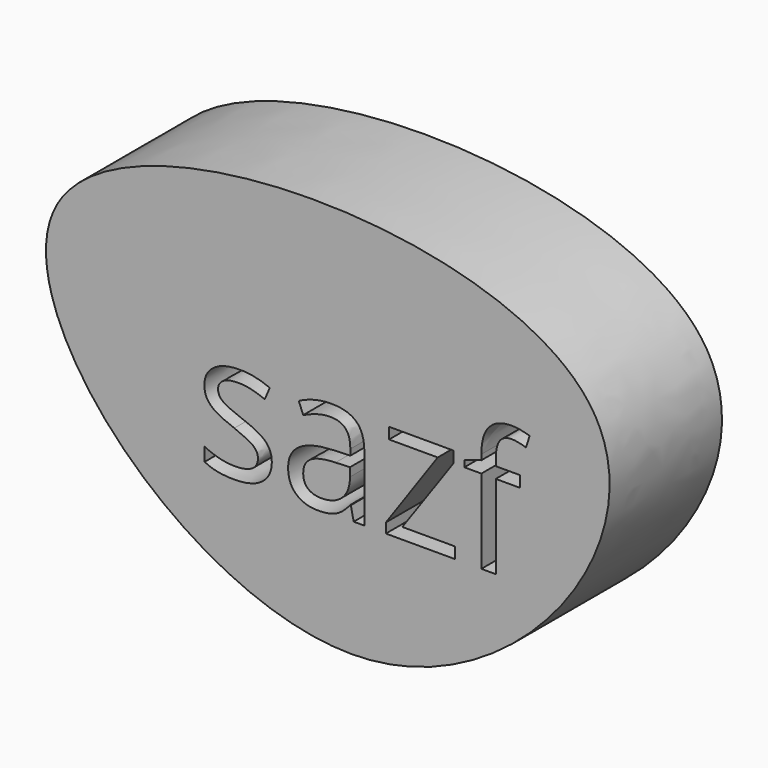
from build123d import *

# Parameters (mm, degrees)
F1_DEPTH     = 25
F2_TEXT_SIZE = 31.6207856587
F3_DEPTH     = 25.0010001


# Not quite as in the source:
# - Text() gives the source's letters only with a copy of the font that has no kerning and outlines rounded to 1/6400 em; it was checked with that copy


with BuildPart() as f1:
    # F0 (on Front) → F1 (new body)
    with BuildSketch(Plane.XZ):
        with BuildLine():
            add(Edge.make_bspline(
                [(-53.528226912, 33.931452781), (-64.31178653, 15.1914120234), (1.5680303917, -54.136069047), (84.1193518361, 54.304890427), (-41.4424797782, 54.9344797865), (-53.528226912, 33.931452781)],
                knots=[0, 0, 0, 0, 0.3267031824, 0.633845206, 1, 1, 1, 1], degree=3))
        make_face()
    extrude(amount=F1_DEPTH)

    # F2 (on face) → F3 (cut, through all)
    with BuildSketch(Plane.XZ.offset(25)):
        with Locations((-29.0093850344, 1.2577723246)):
            Text('sazf', F2_TEXT_SIZE, font='Open Sans', text_align=(TextAlign.LEFT, TextAlign.BOTTOM))
    extrude(amount=-F3_DEPTH, mode=Mode.SUBTRACT)


solid = f1.part
